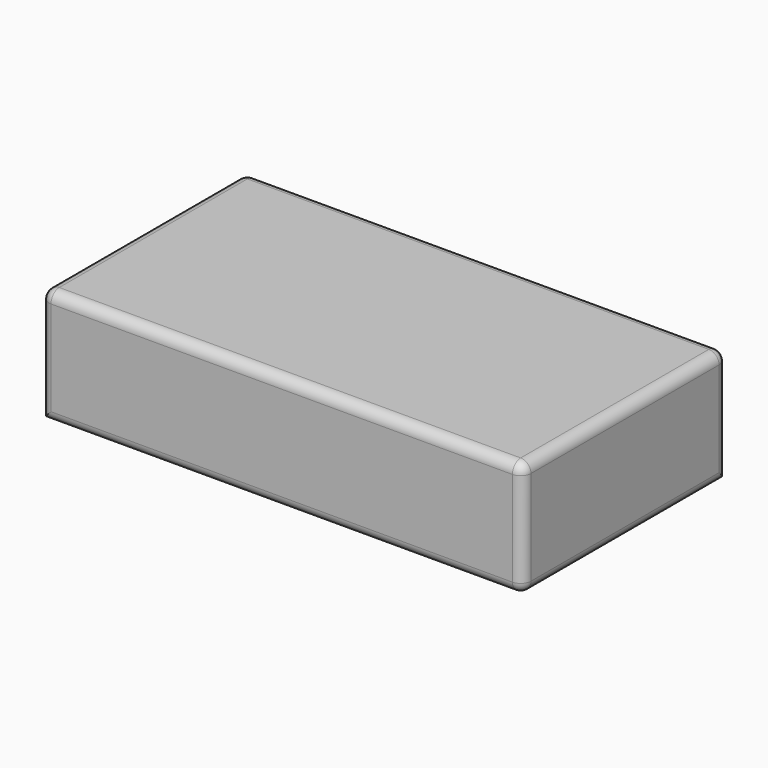
from build123d import *

# Parameters (mm, degrees)
F0_W        = 237.6048713923
F0_H        = 126.0424219072
F1_DEPTH    = 56.896
F2_R        = 5.08
F3_T1_DEPTH = 64.516
F3_S5_W     = 5.08
F3_S5_H     = 5.08
F3_T6_DEPTH = 5.08


# Not quite as in the source:
# - a fillet or chamfer that OpenCascade refuses, or shapes differently, is made with other operations: its cross-section is extruded or revolved along the edge and cut away or added


with BuildPart() as f1:
    # F0 (on Top) → F1 (new body)
    with BuildSketch(Plane.XY):
        with Locations((-7.780559361, 5.7301688939)):
            Rectangle(F0_W, F0_H)
    extrude(amount=F1_DEPTH)

    # F2
    f2_edges = [f1.edges().sort_by_distance(p)[0] for p in [
        (-7.780559, -57.291042, 56.896),
        (-126.582995, 5.730169, 56.896),
        (-7.780559, 68.75138, 56.896),
        (111.021876, 5.730169, 56.896),
        (111.021876, 68.75138, 28.448),
        (111.021876, -57.291042, 28.448),
        (111.021876, 5.730169, 0),
        (-7.780559, -57.291042, 0),
        (-126.582995, -57.291042, 28.448),
    ]]
    fillet(f2_edges, radius=F2_R)

    # F3: fillet of radius 5.08 on 1 edges, made by hand

    # F3_s2 → F3_t1 (cut)
    with BuildSketch(Plane.XY.offset(-12.7)):
        with BuildLine():
            ThreePointArc((-121.5029950571, 68.7513798475), (-125.0950975055, 67.263482296), (-126.5829950571, 63.6713798475))
            Line((-126.5829950571, 63.6713798475), (-126.5829950571, 68.7513798475))
            Line((-126.5829950571, 68.7513798475), (-121.5029950571, 68.7513798475))
        make_face()
    extrude(amount=F3_T1_DEPTH, mode=Mode.SUBTRACT)


with BuildPart() as f3_tool4:
    # F3_s5 → F3_t6 (new body)
    with BuildSketch(Plane.XZ.offset(-63.6713798475)):
        with Locations((-124.0429950571, 54.356)):
            Rectangle(F3_S5_W, F3_S5_H)
    extrude(amount=-F3_T6_DEPTH)

    # F3_s7 → F3_t8 (revolve, cut)
    with BuildSketch(Plane(origin=(-121.5029950571, 63.6713798475, 51.816), x_dir=(0.7071067812, 0, -0.7071067812), z_dir=(0.7071067812, 0, 0.7071067812))):
        with BuildLine():
            ThreePointArc((0, -5.08), (5.08, 0), (0, 5.08))
            Line((0, 5.08), (0, -5.08))
        make_face()
    revolve(axis=Axis((-121.5029950571, 63.6713798475, 51.816), (0, 1, 0)), mode=Mode.SUBTRACT)


with BuildPart() as f1_1:
    add(f1.part)

    # F3_t3: cut F3_tool4
    add(f3_tool4.part, mode=Mode.SUBTRACT)


solid = f1_1.part
